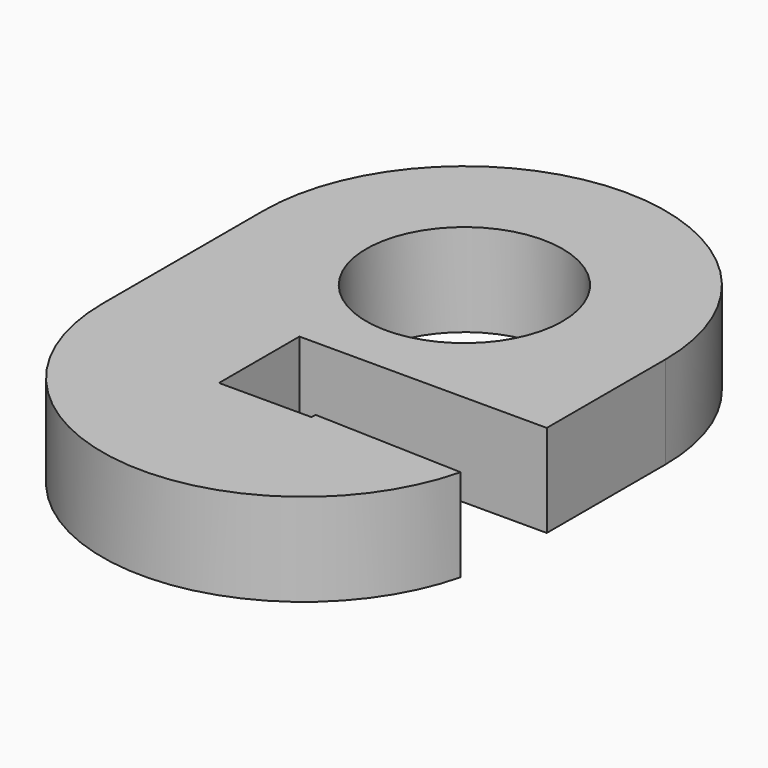
from build123d import *

# Parameters (mm, degrees)
F0_R     = 6.1976
F1_DEPTH = 5.842
F3_DEPTH = 5.842


# Not quite as in the source:
# - a feature names something its author has since deleted; it is built from what else it names


with BuildPart() as f1:
    # F0 (on Top) → F1 (new body)
    with BuildSketch(Plane.XY):
        with BuildLine():
            ThreePointArc((-12.7, 0), (0, -12.7), (12.7, 0))
            ThreePointArc((12.7, 0), (0, 12.7), (-12.7, 0))
        make_face()
        Circle(F0_R, mode=Mode.SUBTRACT)
        with BuildLine():
            Line((12.7, -12.7), (12.7, 0))
            ThreePointArc((12.7, 0), (0, -12.7), (-12.7, 0))
            Line((-12.7, 0), (-12.7, -12.7))
            ThreePointArc((-12.7, -12.7), (0, -25.4), (12.7, -12.7))
        make_face()
    extrude(amount=-F1_DEPTH)

    # F2 (on face) → F3 (cut, through all)
    with BuildSketch(Plane.XY):
        with BuildLine():
            Line((12.7, -9.3726), (-2.921, -9.3726))
            Line((-2.921, -9.3726), (-2.921, -15.7226))
            Line((-2.921, -15.7226), (2.921, -15.7226))
            Line((2.921, -15.7226), (2.921, -15.4051))
            Line((2.921, -15.4051), (12.3350674599, -15.7226))
            ThreePointArc((12.3350674599, -15.7226), (12.6084367933, -14.2222751491), (12.7, -12.7))
            Line((12.7, -12.7), (12.7, -9.3726))
        make_face()
    extrude(amount=-F3_DEPTH, mode=Mode.SUBTRACT)


solid = f1.part
